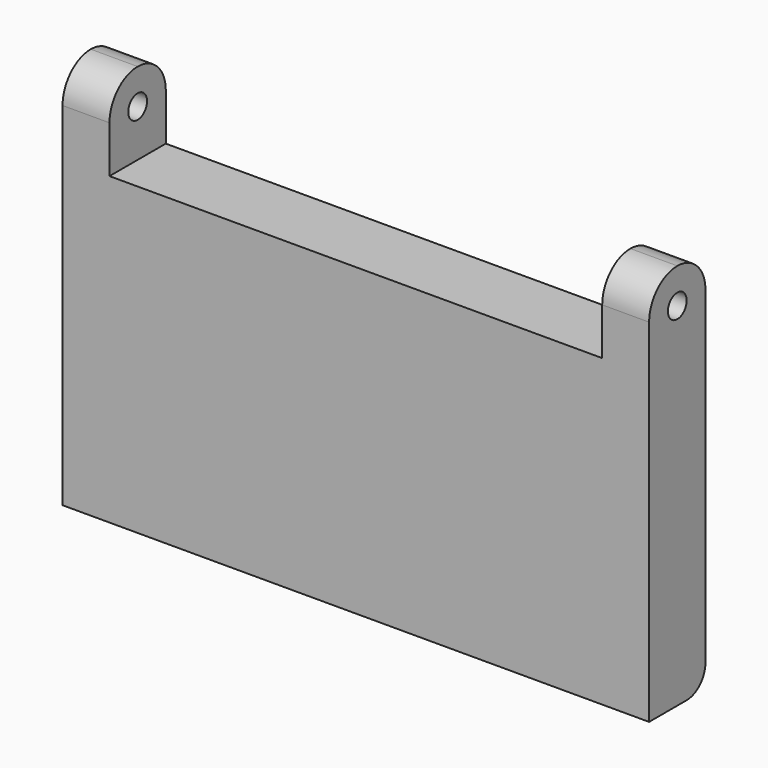
from build123d import *

# Parameters (mm, degrees)
F1_DEPTH = 15
F2_R     = 2.5
F3_DEPTH = 125.001
F4_R     = 7.49999
F5_R     = 5


# Not quite as in the source:
# - a fillet or chamfer is up to 0.001 mm smaller than in the source, because OpenCascade refuses the exact size


with BuildPart() as f1:
    # F0 (on Front) → F1 (new body)
    with BuildSketch(Plane.XZ):
        Polygon((-62.5, 23.75), (-62.5, -41.25), (62.5, -41.25), (62.5, 23.75), (62.5, 41.25), (52.5, 41.25), (52.5, 23.75), (-52.5, 23.75), (-52.5, 41.25), (-62.5, 41.25), align=None)
    extrude(amount=F1_DEPTH)

    # F2 (on face) → F3 (cut, through all)
    with BuildSketch(Plane.YZ.offset(62.5)):
        with Locations((-7.5, 33.75)):
            Circle(F2_R)
    extrude(amount=-F3_DEPTH, mode=Mode.SUBTRACT)

    # F4 (radius 7.5 in the source; OpenCascade refuses exactly that, so slightly less here)
    f4_edges = [f1.edges().sort_by_distance(p)[0] for p in [
        (57.5, 0, 41.25),
        (57.5, -15, 41.25),
        (-57.5, -15, 41.25),
        (-57.5, 0, 41.25),
    ]]
    fillet(f4_edges, radius=F4_R)

    # F5
    f5_edges = [f1.edges().sort_by_distance(p)[0] for p in [
        (0, 0, -41.25),
    ]]
    fillet(f5_edges, radius=F5_R)


solid = f1.part
